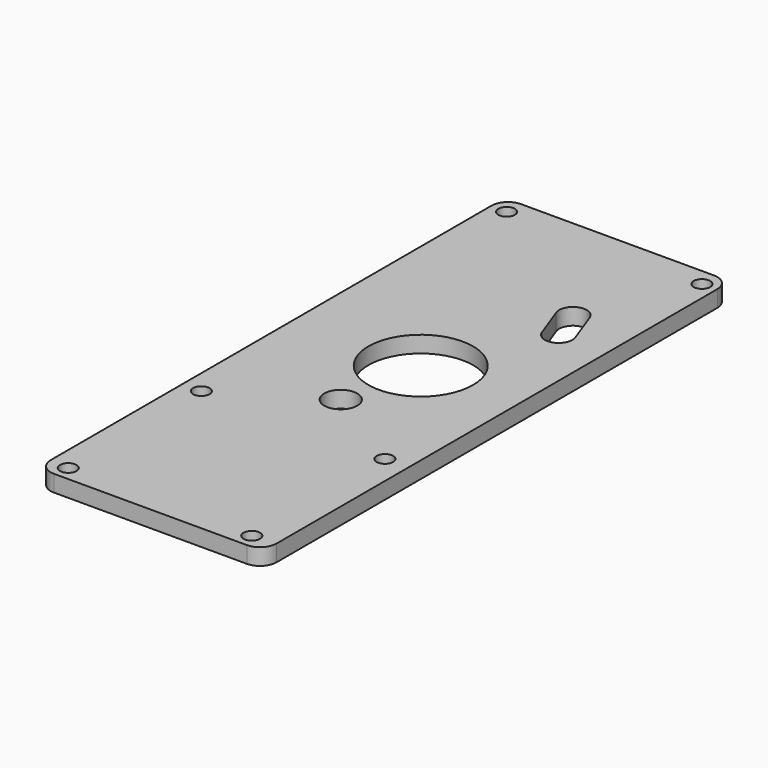
from build123d import *

# Parameters (mm, degrees)
F0_W     = 41
F0_H     = 106
F0_R     = 1.5
F0_R_2   = 5.05
F0_R_3   = 2
F0_R_4   = 3
F0_R_5   = 9.5
F1_DEPTH = 3
F2_R     = 3


# Not quite as in the source:
# - a feature names something its author has since deleted; it is built from what else it names


with BuildPart() as f1:
    # F0 (on Top) → F1 (new body)
    with BuildSketch(Plane.XY):
        with Locations((-1.1801278293, -1.1353523731)):
            Rectangle(F0_W, F0_H)
        with Locations((-18.2301278293, -51.4703523731)):
            Circle(F0_R, mode=Mode.SUBTRACT)
        with Locations((-6.776117335, -33.481924504)):
            Circle(F0_R_2, mode=Mode.SUBTRACT)
        with Locations((-18.2301278293, -21.2703523731)):
            Circle(F0_R, mode=Mode.SUBTRACT)
        with Locations((-11.8353097141, -18.4490393624)):
            Circle(F0_R_3, mode=Mode.SUBTRACT)
        with BuildLine():
            ThreePointArc((0.9913514778, -28.481924504), (-4.9415118708, -25.855220261), (-8.0481067447, -20.1589485871))
            Line((-8.0481067447, -20.1589485871), (9.9913514778, -20.516399593))
            Line((9.9913514778, -20.516399593), (9.9913514778, -46.516399593))
            Line((9.9913514778, -46.516399593), (-8.0481067447, -46.804900421))
            ThreePointArc((-8.0481067447, -46.804900421), (-4.9415118708, -41.1086287471), (0.9913514778, -38.481924504))
            Line((0.9913514778, -38.481924504), (0.9913514778, -28.481924504))
        make_face(mode=Mode.SUBTRACT)
        with Locations((15.0892422113, -51.4703523731)):
            Circle(F0_R, mode=Mode.SUBTRACT)
        with Locations((-1.1801278293, -10.9442314133)):
            Circle(F0_R_4, mode=Mode.SUBTRACT)
        with Locations((15.0892422113, -21.2703523731)):
            Circle(F0_R, mode=Mode.SUBTRACT)
        with Locations((-11.8353097141, -0.1353523731)):
            Circle(F0_R_3, mode=Mode.SUBTRACT)
        with Locations((-11.8353097141, 18.1783346161)):
            Circle(F0_R_3, mode=Mode.SUBTRACT)
        with Locations((-18.8301271707, 48.7366476269)):
            Circle(F0_R, mode=Mode.SUBTRACT)
        with Locations((-6.776117335, 33.2112197578)):
            Circle(F0_R_2, mode=Mode.SUBTRACT)
        with Locations((1.1698721707, 4.2646476269)):
            Circle(F0_R_5, mode=Mode.SUBTRACT)
        with BuildLine():
            ThreePointArc((0.9913514778, 38.2112197578), (-4.9415118708, 40.8379240009), (-8.0481067447, 46.5341956747))
            Line((-8.0481067447, 46.5341956747), (9.9913514778, 46.2456948468))
            Line((9.9913514778, 46.2456948468), (9.9913514778, 31.7237218389))
            ThreePointArc((9.9913514778, 31.7237218389), (10.4081379557, 31.2391097076), (10.6884153726, 30.6646495649))
            Line((10.6884153726, 30.6646495649), (12.8669505005, 24.7255908967))
            ThreePointArc((12.8669505005, 24.7255908967), (12.9813448828, 24.3018570593), (13.0198721707, 23.8646476269))
            ThreePointArc((13.0198721707, 23.8646476269), (12.0896967258, 21.9189727141), (9.9913514778, 21.4211530234))
            Line((9.9913514778, 21.4211530234), (9.9913514778, 20.2456948468))
            Line((9.9913514778, 20.2456948468), (-8.0481067447, 19.8882438409))
            ThreePointArc((-8.0481067447, 19.8882438409), (-4.9415118708, 25.5845155147), (0.9913514778, 28.2112197578))
            Line((0.9913514778, 28.2112197578), (0.9913514778, 38.2112197578))
        make_face(mode=Mode.SUBTRACT)
        with Locations((16.6392421771, 48.7366476269)):
            Circle(F0_R, mode=Mode.SUBTRACT)
        with BuildLine():
            Line((9.9913514778, -20.516399593), (-8.0481067447, -20.1589485871))
            ThreePointArc((-8.0481067447, -20.1589485871), (-4.9415118708, -25.855220261), (0.9913514778, -28.481924504))
            Line((0.9913514778, -28.481924504), (0.9913514778, -38.481924504))
            ThreePointArc((0.9913514778, -38.481924504), (-4.9415118708, -41.1086287471), (-8.0481067447, -46.804900421))
            Line((-8.0481067447, -46.804900421), (9.9913514778, -46.516399593))
            Line((9.9913514778, -46.516399593), (9.9913514778, -20.516399593))
        make_face()
        with Locations((-2.2937730764, -41.981924504)):
            Circle(F0_R, mode=Mode.SUBTRACT)
        with Locations((-2.2937730764, -24.981924504)):
            Circle(F0_R, mode=Mode.SUBTRACT)
        with BuildLine():
            Line((9.9913514778, 46.2456948468), (-8.0481067447, 46.5341956747))
            ThreePointArc((-8.0481067447, 46.5341956747), (-4.9415118708, 40.8379240009), (0.9913514778, 38.2112197578))
            Line((0.9913514778, 38.2112197578), (0.9913514778, 28.2112197578))
            ThreePointArc((0.9913514778, 28.2112197578), (-4.9415118708, 25.5845155147), (-8.0481067447, 19.8882438409))
            Line((-8.0481067447, 19.8882438409), (9.9913514778, 20.2456948468))
            Line((9.9913514778, 20.2456948468), (9.9913514778, 21.4211530234))
            ThreePointArc((9.9913514778, 21.4211530234), (8.9707387909, 21.9024586015), (8.2657292668, 22.7835186943))
            ThreePointArc((8.2657292668, 22.7835186943), (8.1741724057, 22.9999554201), (8.1033430916, 23.2240329142))
            Line((8.1033430916, 23.2240329142), (5.9741724057, 28.9999554201))
            ThreePointArc((5.9741724057, 28.9999554201), (6.9168863609, 31.9338578186), (9.9913514778, 31.7237218389))
            Line((9.9913514778, 31.7237218389), (9.9913514778, 46.2456948468))
        make_face()
        with Locations((-2.2937730764, 24.7112197578)):
            Circle(F0_R, mode=Mode.SUBTRACT)
        with Locations((-2.2937730764, 41.7112197578)):
            Circle(F0_R, mode=Mode.SUBTRACT)
        with Locations((-6.776117335, 33.2112197578)):
            Circle(F0_R_2)
        with Locations((-6.776117335, -33.481924504)):
            Circle(F0_R_2)
        with Locations((-11.8353097141, -18.4490393624)):
            Circle(F0_R_3)
        with Locations((-11.8353097141, -0.1353523731)):
            Circle(F0_R_3)
        with Locations((-11.8353097141, 18.1783346161)):
            Circle(F0_R_3)
        with Locations((-2.2937730764, -24.981924504)):
            Circle(F0_R)
        with Locations((-2.2937730764, -41.981924504)):
            Circle(F0_R)
        with Locations((-2.2937730764, 24.7112197578)):
            Circle(F0_R)
        with Locations((-2.2937730764, 41.7112197578)):
            Circle(F0_R)
    extrude(amount=F1_DEPTH)

    # F2
    f2_edges = [f1.edges().sort_by_distance(p)[0] for p in [
        (-21.680128, 51.864648, 1.5),
        (-21.680128, -54.135352, 1.5),
        (19.319872, -54.135352, 1.5),
        (19.319872, 51.864648, 1.5),
    ]]
    fillet(f2_edges, radius=F2_R)


solid = f1.part
